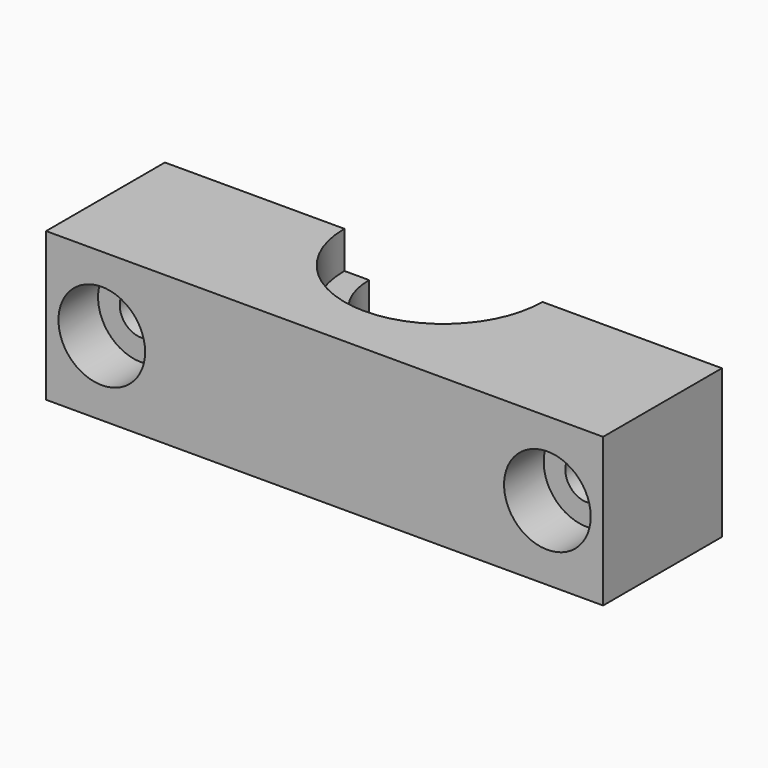
from build123d import *

# Parameters (mm, degrees)
F0_W     = 45
F0_H     = 12
F0_R     = 3.5
F0_R_2   = 1.75
F1_DEPTH = 12
F2_DEPTH = 4
F4_DEPTH = 12.001
F3_R     = 8
F3_R_2   = 6
F5_DEPTH = 3
F6_R     = 8
F7_DEPTH = 3


with BuildPart() as f1:
    # F0 (on Front) → F1 (new body)
    with BuildSketch(Plane.XZ):
        Rectangle(F0_W, F0_H)
        with Locations((-18, 0)):
            Circle(F0_R, mode=Mode.SUBTRACT)
        with Locations((18, 0)):
            Circle(F0_R, mode=Mode.SUBTRACT)
        with Locations((-18, 0)):
            Circle(F0_R)
        with Locations((-18, 0)):
            Circle(F0_R_2, mode=Mode.SUBTRACT)
        with Locations((18, 0)):
            Circle(F0_R)
        with Locations((18, 0)):
            Circle(F0_R_2, mode=Mode.SUBTRACT)
    extrude(amount=-F1_DEPTH)

    # F0 (on Front) → F2 (cut)
    with BuildSketch(Plane.XZ):
        with Locations((-18, 0)):
            Circle(F0_R)
        with Locations((-18, 0)):
            Circle(F0_R_2, mode=Mode.SUBTRACT)
        with Locations((18, 0)):
            Circle(F0_R)
        with Locations((18, 0)):
            Circle(F0_R_2, mode=Mode.SUBTRACT)
    extrude(amount=-F2_DEPTH, mode=Mode.SUBTRACT)

    # F3 (on face) → F4 (cut, through all)
    with BuildSketch(Plane.XY.offset(6)):
        with BuildLine():
            Line((-6, 12), (6, 12))
            ThreePointArc((6, 12), (0, 18), (-6, 12))
        make_face()
        with BuildLine():
            ThreePointArc((-6, 12), (0, 6), (6, 12))
            Line((6, 12), (-6, 12))
        make_face()
    extrude(amount=-F4_DEPTH, mode=Mode.SUBTRACT)

    # F3 (on face) → F5 (cut)
    with BuildSketch(Plane.XY.offset(6)):
        with Locations((0, 12)):
            Circle(F3_R)
        with Locations((0, 12)):
            Circle(F3_R_2, mode=Mode.SUBTRACT)
    extrude(amount=-F5_DEPTH, mode=Mode.SUBTRACT)

    # F6 (on face) → F7 (cut)
    with BuildSketch(Plane(origin=(0, 0, -6), x_dir=(1, 0, 0), z_dir=(0, 0, -1))):
        with Locations((0, -12)):
            Circle(F6_R)
    extrude(amount=-F7_DEPTH, mode=Mode.SUBTRACT)


solid = f1.part
